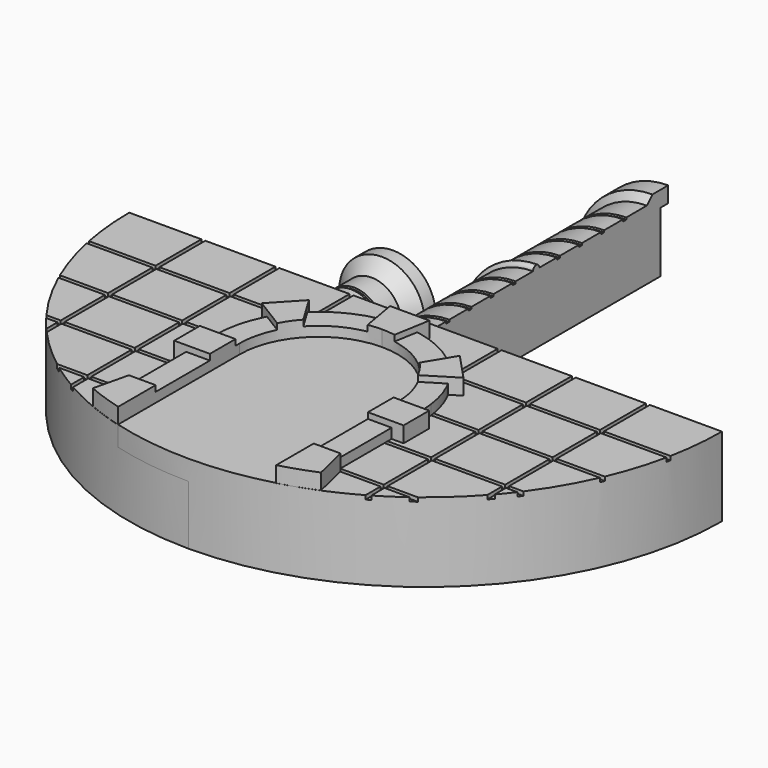
from build123d import *
from build123d import SkipClean  # not in build123d's __all__

# Parameters (mm, degrees)
F1_DEPTH  = 40
F2_W      = 36.5
F2_H      = 2
F2_W_2    = 1.9996949486
F2_W_3    = 35.5003050514
F2_W_4    = 1.9997029738
F2_W_5    = 35.5002970262
F2_W_6    = 2
F2_W_7    = 35.5
F2_H_2    = 28
F2_H_3    = 29
F2_W_8    = 1
F3_DEPTH  = 2
F5_DEPTH  = 10
F6_W      = 12
F6_H      = 12.1140629053
F6_H_2    = 4.5821502209
F7_DEPTH  = 5
F8_W      = 25.165
F8_H      = 16.205
F9_DEPTH  = 8
F10_R     = 180
F11_DEPTH = 114
F12_DEPTH = 25
F14_DEPTH = 10.1
F17_ANGLE = 90
F19_ANGLE = 180


with BuildPart() as f1:
    # F0 (on Top) → F1 (new body)
    with BuildSketch(Plane.XY):
        with BuildLine():
            Line((0, -145.5492973328), (-150, -145.5492973328))
            ThreePointArc((-150, -145.5492973328), (-106.066017178, -251.6153145107), (0, -295.5492973328))
            Line((0, -295.5492973328), (0, -145.5492973328))
        make_face()
    extrude(amount=F1_DEPTH)

    # F2 (on face) → F3 (cut)
    with BuildSketch(Plane.XY.offset(40)):
        with Locations((-131.75, -265.5492973328)):
            Rectangle(F2_W, F2_H)
        Polygon((-111.5003050514, -266.5492973328), (-113.5, -266.5492973328), (-113.5, -295.5492973328), (-111.5003050514, -295.5491274107), align=None)
        with Locations((-112.5001525257, -175.5492973328)):
            Rectangle(F2_W_2, F2_H)
        with Locations((-93.7501525257, -175.5492973328)):
            Rectangle(F2_W_3, F2_H)
        with Locations((-75.0001485131, -175.5492973328)):
            Rectangle(F2_W_4, F2_H)
        with Locations((-56.2501485131, -175.5492973328)):
            Rectangle(F2_W_5, F2_H)
        with Locations((-37.5, -175.5492973328)):
            Rectangle(F2_W_6, F2_H)
        with Locations((-18.75, -175.5492973328)):
            Rectangle(F2_W_7, F2_H)
        with Locations((-112.5001525257, -190.5492973328)):
            Rectangle(F2_W_2, F2_H_2)
        with Locations((-112.5001525257, -205.5492973328)):
            Rectangle(F2_W_2, F2_H)
        with Locations((-112.5001525257, -220.5492973328)):
            Rectangle(F2_W_2, F2_H_2)
        with Locations((-112.5001525257, -265.5492973328)):
            Rectangle(F2_W_2, F2_H)
        with Locations((-75.0001485131, -265.5492973328)):
            Rectangle(F2_W_4, F2_H)
        with Locations((-56.2501485131, -265.5492973328)):
            Rectangle(F2_W_5, F2_H)
        with Locations((-37.5, -265.5492973328)):
            Rectangle(F2_W_6, F2_H)
        with Locations((-18.75, -265.5492973328)):
            Rectangle(F2_W_7, F2_H)
        with BuildLine():
            Line((-147.1699697629, -174.5492973328), (-150, -174.5492973328))
            Line((-150, -174.5492973328), (-150, -176.5492973328))
            Line((-150, -176.5492973328), (-146.7617116281, -176.5492973328))
            ThreePointArc((-146.7617116281, -176.5492973328), (-146.9692428072, -175.5499918027), (-147.1699697629, -174.5492973328))
        make_face()
        with BuildLine():
            ThreePointArc((-137.0364914904, -206.5492973328), (-137.4765780481, -205.5508847133), (-137.9093905432, -204.5492973328))
            Line((-137.9093905432, -204.5492973328), (-150, -204.5492973328))
            Line((-150, -204.5492973328), (-150, -206.5492973328))
            Line((-150, -206.5492973328), (-137.0364914904, -206.5492973328))
        make_face()
        with BuildLine():
            ThreePointArc((-119.2434484573, -236.5492973328), (-119.9976559728, -235.5524226176), (-120.7435298474, -234.5492973328))
            Line((-120.7435298474, -234.5492973328), (-150, -234.5492973328))
            Line((-150, -234.5492973328), (-150, -236.5492973328))
            Line((-150, -236.5492973328), (-119.2434484573, -236.5492973328))
        make_face()
        Polygon((-38.5, -140.4211074114), (-38.5, -145.5492973328), (-36.5, -145.5492973328), (-36.5, -139.0285342932), align=None)
        with BuildLine():
            ThreePointArc((-36.5, -291.0407060138), (-37.5008889233, -290.7859432936), (-38.5, -290.5242951772))
            Line((-38.5, -290.5242951772), (-38.5, -295.5492973328))
            Line((-38.5, -295.5492973328), (-36.5, -295.5492973328))
            Line((-36.5, -295.5492973328), (-36.5, -291.0407060138))
        make_face()
        Polygon((-76, -139.307051897), (-76, -145.5492973328), (-74.0002970262, -145.5492973328), (-74.0002970262, -139.0285756567), align=None)
        with BuildLine():
            ThreePointArc((-74.0002970262, -276.0251803152), (-75.0023702252, -275.4517394214), (-76, -274.8706026154))
            Line((-76, -274.8706026154), (-76, -295.5492973328))
            Line((-76, -295.5492973328), (-74.0002970262, -295.5493386963))
            Line((-74.0002970262, -295.5493386963), (-74.0002970262, -276.0251803152))
        make_face()
        Polygon((-113.5, -139.307051897), (-113.5, -145.5492973328), (-111.5003050514, -145.5492973328), (-111.5003050514, -140.4209374893), align=None)
        with BuildLine():
            ThreePointArc((-111.5003050514, -245.8871365234), (-112.5058662775, -244.7583193678), (-113.5, -243.6194253025))
            Line((-113.5, -243.6194253025), (-113.5, -264.5492973328))
            Line((-113.5, -264.5492973328), (-111.5003050514, -264.5492973328))
            Line((-111.5003050514, -264.5492973328), (-111.5003050514, -245.8871365234))
        make_face()
        with BuildLine():
            Line((-91.3181252545, -264.5492973328), (-111.5003050514, -264.5492973328))
            Line((-111.5003050514, -264.5492973328), (-111.5003050514, -266.5492973328))
            Line((-111.5003050514, -266.5492973328), (-88.6510011224, -266.5492973328))
            ThreePointArc((-88.6510011224, -266.5492973328), (-89.9901195255, -265.5567070531), (-91.3181252545, -264.5492973328))
        make_face()
        with BuildLine():
            Line((-113.5, -174.5492973328), (-147.1699697629, -174.5492973328))
            ThreePointArc((-147.1699697629, -174.5492973328), (-146.9692428072, -175.5499918027), (-146.7617116281, -176.5492973328))
            Line((-146.7617116281, -176.5492973328), (-113.5, -176.5492973328))
            Line((-113.5, -176.5492973328), (-113.5, -174.5492973328))
        make_face()
        with Locations((-112.5001525257, -160.0492973328)):
            Rectangle(F2_W_2, F2_H_3)
        with Locations((-75.0001485131, -160.0492973328)):
            Rectangle(F2_W_4, F2_H_3)
        with Locations((-37.5, -160.0492973328)):
            Rectangle(F2_W_6, F2_H_3)
        with Locations((-0.5, -175.5492973328)):
            Rectangle(F2_W_8, F2_H)
        with Locations((-0.5, -190.5492973328)):
            Rectangle(F2_W_8, F2_H_2)
        with BuildLine():
            Line((-113.5, -204.5492973328), (-137.9093905432, -204.5492973328))
            ThreePointArc((-137.9093905432, -204.5492973328), (-137.4765780481, -205.5508847133), (-137.0364914904, -206.5492973328))
            Line((-137.0364914904, -206.5492973328), (-113.5, -206.5492973328))
            Line((-113.5, -206.5492973328), (-113.5, -204.5492973328))
        make_face()
        with Locations((-0.5, -205.5492973328)):
            Rectangle(F2_W_8, F2_H)
        with Locations((-0.5, -220.5492973328)):
            Rectangle(F2_W_8, F2_H_2)
        with BuildLine():
            Line((-113.5, -234.5492973328), (-120.7435298474, -234.5492973328))
            ThreePointArc((-120.7435298474, -234.5492973328), (-119.9976559728, -235.5524226176), (-119.2434484573, -236.5492973328))
            Line((-119.2434484573, -236.5492973328), (-113.5, -236.5492973328))
            Line((-113.5, -236.5492973328), (-113.5, -234.5492973328))
        make_face()
        with Locations((-0.5, -235.5492973328)):
            Rectangle(F2_W_8, F2_H)
        with BuildLine():
            Line((-111.5003050514, -236.5492973328), (-113.5, -236.5492973328))
            Line((-113.5, -236.5492973328), (-113.5, -243.6194253025))
            ThreePointArc((-113.5, -243.6194253025), (-112.5058662775, -244.7583193678), (-111.5003050514, -245.8871365234))
            Line((-111.5003050514, -245.8871365234), (-111.5003050514, -236.5492973328))
        make_face()
        with Locations((-0.5, -250.5492973328)):
            Rectangle(F2_W_8, F2_H_2)
        with BuildLine():
            Line((-76, -264.5492973328), (-91.3181252545, -264.5492973328))
            ThreePointArc((-91.3181252545, -264.5492973328), (-89.9901195255, -265.5567070531), (-88.6510011224, -266.5492973328))
            Line((-88.6510011224, -266.5492973328), (-76, -266.5492973328))
            Line((-76, -266.5492973328), (-76, -264.5492973328))
        make_face()
        with Locations((-0.5, -265.5492973328)):
            Rectangle(F2_W_8, F2_H)
        with BuildLine():
            Line((-74.0002970262, -266.5492973328), (-76, -266.5492973328))
            Line((-76, -266.5492973328), (-76, -274.8706026154))
            ThreePointArc((-76, -274.8706026154), (-75.0023702252, -275.4517394214), (-74.0002970262, -276.0251803152))
            Line((-74.0002970262, -276.0251803152), (-74.0002970262, -266.5492973328))
        make_face()
        with BuildLine():
            Line((-36.5, -266.5492973328), (-38.5, -266.5492973328))
            Line((-38.5, -266.5492973328), (-38.5, -290.5242951772))
            ThreePointArc((-38.5, -290.5242951772), (-37.5008889233, -290.7859432936), (-36.5, -291.0407060138))
            Line((-36.5, -291.0407060138), (-36.5, -266.5492973328))
        make_face()
        with Locations((-0.5, -160.0492973328)):
            Rectangle(F2_W_8, F2_H_3)
        with BuildLine():
            Line((-1, -266.5492973328), (-1, -295.5459639624))
            ThreePointArc((-1, -295.5459639624), (-0.5000027778, -295.5484639879), (0, -295.5492973328))
            Line((0, -295.5492973328), (0, -266.5492973328))
            Line((0, -266.5492973328), (-1, -266.5492973328))
        make_face()
        with BuildLine():
            Line((0, -145.5492973328), (0, -174.5492973328))
            Line((0, -174.5492973328), (0, -176.5492973328))
            Line((0, -176.5492973328), (0, -204.5492973328))
            Line((0, -204.5492973328), (0, -206.5492973328))
            Line((0, -206.5492973328), (0, -234.5492973328))
            Line((0, -234.5492973328), (0, -236.5492973328))
            Line((0, -236.5492973328), (0, -264.5492973328))
            Line((0, -264.5492973328), (0, -266.5492973328))
            Line((0, -266.5492973328), (0, -295.5492973328))
            ThreePointArc((0, -295.5492973328), (-0.5000027778, -295.5484639879), (-1, -295.5459639624))
            Line((-1, -295.5459639624), (-1, -302.514731884))
            Line((-1, -302.514731884), (2.084, -302.514731884))
            Line((2.084, -302.514731884), (2.084, -140.6996101141))
            Line((2.084, -140.6996101141), (-1, -140.6996101141))
            Line((-1, -140.6996101141), (-1, -145.5492973328))
            Line((-1, -145.5492973328), (0, -145.5492973328))
        make_face()
        with Locations((-75.0001485131, -190.5492973328)):
            Rectangle(F2_W_4, F2_H_2)
        with Locations((-93.7501525257, -205.5492973328)):
            Rectangle(F2_W_3, F2_H)
        with Locations((-56.2501485131, -205.5492973328)):
            Rectangle(F2_W_5, F2_H)
        with Locations((-37.5, -190.5492973328)):
            Rectangle(F2_W_6, F2_H_2)
        with Locations((-18.75, -205.5492973328)):
            Rectangle(F2_W_7, F2_H)
        with Locations((-18.75, -235.5492973328)):
            Rectangle(F2_W_7, F2_H)
        with Locations((-56.2501485131, -235.5492973328)):
            Rectangle(F2_W_5, F2_H)
        with Locations((-37.5, -220.5492973328)):
            Rectangle(F2_W_6, F2_H_2)
        with Locations((-37.5, -250.5492973328)):
            Rectangle(F2_W_6, F2_H_2)
        with Locations((-75.0001485131, -250.5492973328)):
            Rectangle(F2_W_4, F2_H_2)
        with Locations((-93.7501525257, -235.5492973328)):
            Rectangle(F2_W_3, F2_H)
        with Locations((-75.0001485131, -220.5492973328)):
            Rectangle(F2_W_4, F2_H_2)
        with Locations((-112.5001525257, -235.5492973328)):
            Rectangle(F2_W_2, F2_H)
        with Locations((-75.0001485131, -205.5492973328)):
            Rectangle(F2_W_4, F2_H)
        with Locations((-75.0001485131, -235.5492973328)):
            Rectangle(F2_W_4, F2_H)
        with Locations((-37.5, -205.5492973328)):
            Rectangle(F2_W_6, F2_H)
        with Locations((-37.5, -235.5492973328)):
            Rectangle(F2_W_6, F2_H)
    extrude(amount=-F3_DEPTH, mode=Mode.SUBTRACT)

    # F4 (on face) → F5 (cut)
    with BuildSketch(Plane.XY.offset(40)):
        with BuildLine():
            ThreePointArc((0, -173.1574415227), (-28.2842712475, -184.8731702752), (-40, -213.1574415227))
            Line((-40, -213.1574415227), (-40, -295.5492973328))
            Line((-40, -295.5492973328), (0, -300.0960052013))
            Line((0, -300.0960052013), (0, -173.1574415227))
        make_face()
    extrude(amount=-F5_DEPTH, mode=Mode.SUBTRACT)

    # F6 (on face) → F7 (join)
    with BuildSketch(Plane.XY.offset(40)):
        with Locations((-46, -223.9101156592)):
            Rectangle(F6_W, F6_H)
        with BuildLine():
            ThreePointArc((-46.8565880337, -190.6083803928), (-49.8587047828, -198.3889088474), (-51.5784105064, -206.5492973328))
            Line((-51.5784105064, -206.5492973328), (-39.4503793437, -206.5492973328))
            ThreePointArc((-39.4503793437, -206.5492973328), (-38.1943316303, -201.274974131), (-36.2365551908, -196.2189626092))
            Line((-36.2365551908, -196.2189626092), (-46.8565880337, -190.6083803928))
        make_face()
        with BuildLine():
            Line((-30.020735185, -186.7234584904), (-38.3793901323, -178.071512533))
            ThreePointArc((-38.3793901323, -178.071512533), (-43.0765163101, -184.0298988425), (-46.8565880337, -190.6083803928))
            Line((-46.8565880337, -190.6083803928), (-36.2365551908, -196.2189626092))
            ThreePointArc((-36.2365551908, -196.2189626092), (-33.467122398, -191.249641122), (-30.020735185, -186.7234584904))
        make_face()
        with BuildLine():
            Line((-8.9829999717, -174.1791692225), (-10.5112668126, -162.2308937309))
            ThreePointArc((-10.5112668126, -162.2308937309), (-25.6964080201, -167.9502007878), (-38.3793901323, -178.071512533))
            Line((-38.3793901323, -178.071512533), (-30.020735185, -186.7234584904))
            ThreePointArc((-30.020735185, -186.7234584904), (-20.4856690726, -178.8014032958), (-8.9829999717, -174.1791692225))
        make_face()
        with BuildLine():
            ThreePointArc((0, -173.1574415227), (3.7325532598, -173.3319717055), (7.4325343594, -173.8540392145))
            Line((7.4325343594, -173.8540392145), (7.4325343594, -161.6913611105))
            ThreePointArc((7.4325343594, -161.6913611105), (-1.5628250835, -161.1809316576), (-10.5112668126, -162.2308937309))
            Line((-10.5112668126, -162.2308937309), (-8.9829999717, -174.1791692225))
            ThreePointArc((-8.9829999717, -174.1791692225), (-4.5204594895, -173.413694266), (0, -173.1574415227))
        make_face()
        with BuildLine():
            Line((-52, -213.1574415227), (-52, -217.8530842066))
            Line((-52, -217.8530842066), (-40, -217.8530842066))
            Line((-40, -217.8530842066), (-40, -213.1574415227))
            ThreePointArc((-40, -213.1574415227), (-39.8623580195, -209.841960694), (-39.4503793437, -206.5492973328))
            Line((-39.4503793437, -206.5492973328), (-51.5784105064, -206.5492973328))
            ThreePointArc((-51.5784105064, -206.5492973328), (-51.894495596, -209.8466520649), (-52, -213.1574415227))
        make_face()
        with Locations((-46, -232.2582222223)):
            Rectangle(F6_W, F6_H_2)
        Polygon((-52, -234.5492973328), (-52, -265.6105809421), (-49.5921447873, -260.9722912312), (-40, -263.015726515), (-40, -234.5492973328), align=None)
        Polygon((-52, -265.6105809421), (-52, -296.4901937803), (-46.4878678322, -298.051148653), (-40, -284.9790668817), (-40, -263.015726515), (-49.5921447873, -260.9722912312), align=None)
        with BuildLine():
            Line((-52, -296.4901937803), (-52, -298.9768046448))
            ThreePointArc((-52, -298.9768046448), (-46.0343599341, -300.8710205574), (-40, -302.5333729583))
            Line((-40, -302.5333729583), (-40, -290.1176202808))
            Line((-40, -290.1176202808), (-40, -284.9790668817))
            Line((-40, -284.9790668817), (-46.4878678322, -298.051148653))
            Line((-46.4878678322, -298.051148653), (-52, -296.4901937803))
        make_face()
    extrude(amount=F7_DEPTH)

    # F8 (on face) → F9 (join)
    with BuildSketch(Plane.XY.offset(40)):
        Polygon((3.8162998389, -178.7047982216), (2.9556534719, -155.6107550859), (-9.9540557712, -155.6107550859), (-5.9377001598, -178.7047982216), align=None)
        Polygon((-31.0460235924, -197.7236419916), (-27.0463805646, -190.0721490383), (-38.1758213043, -171.6390103102), (-51.0442368686, -185.3769123554), align=None)
        with Locations((-45.456803869, -223.9208732462)):
            Rectangle(F8_W, F8_H)
        Polygon((-37.5396087766, -293.8241362572), (-35.3737460506, -266.3343260786), (-53.53369434, -266.3343260786), (-59.1982627344, -289.992244055), align=None)
    extrude(amount=F9_DEPTH)

    # F10 (on face) → F11 (cut)
    with BuildSketch(Plane.XY.offset(40)):
        with Locations((0, -145.5100625753)):
            Circle(F10_R)
        with BuildLine():
            Line((0, -313.7147128582), (0, -295.5100625753))
            ThreePointArc((0, -295.5100625753), (-106.066017178, -39.4440453974), (150, -145.5100625753))
            ThreePointArc((150, -145.5100625753), (112.9397266269, -244.2248950446), (20.0717580076, -294.1610784834))
            Line((20.0717580076, -294.1610784834), (19.631, -313.7147128582))
            Line((19.631, -313.7147128582), (0, -313.7147128582))
        make_face(mode=Mode.SUBTRACT)
        with BuildLine():
            Line((23.5480514792, -139.9400085211), (0, -139.9400085211))
            Line((0, -139.9400085211), (0, -295.5100625753))
            ThreePointArc((0, -295.5100625753), (10.0585191206, -295.1724365813), (20.0717580076, -294.1610784834))
            Line((20.0717580076, -294.1610784834), (23.5480514792, -139.9400085211))
        make_face()
        with BuildLine():
            ThreePointArc((20.0717580076, -294.1610784834), (10.0585191206, -295.1724365813), (0, -295.5100625753))
            Line((0, -295.5100625753), (0, -313.7147128582))
            Line((0, -313.7147128582), (19.631, -313.7147128582))
            Line((19.631, -313.7147128582), (20.0717580076, -294.1610784834))
        make_face()
    extrude(amount=F11_DEPTH, mode=Mode.SUBTRACT)

    # F12 (cut): a face of the model
    f12_faces = [f1.faces().sort_by_distance(p)[0] for p in [
        (-18.9909582241, -237.4026324516, 30),
    ]]
    extrude(f12_faces, amount=F12_DEPTH, mode=Mode.SUBTRACT)

    # F13: F1 across plane


with BuildPart() as f1_1:
    add(f1.part, clean=False)
    add(f1.part.mirror(Plane.YZ), clean=False)

    # F14 (add): a face of the model
    f14_faces = [f1_1.faces().sort_by_distance(p)[0] for p in [
        (0, -237.4026324516, 30),
    ]]
    with SkipClean():  # cleaning this boolean's faces spoils the solid; the shape is the same uncleaned
        extrude(f14_faces, amount=F14_DEPTH)

    # F16 (on Top) → F17 (revolve)
    with BuildSketch(Plane.XY):
        with BuildLine():
            Line((-35, -145.5492973328), (0, -145.5492973328))
            Line((0, -145.5492973328), (0, 2.9862365732))
            Line((0, 2.9862365732), (-30.5355339059, 2.9862365732))
            Line((-30.5355339059, 2.9862365732), (-30.5355339059, 7.9862365732))
            Line((-30.5355339059, 7.9862365732), (-38.5355339059, 7.9862365732))
            Line((-38.5355339059, 7.9862365732), (-38.5355339059, -2.0137634268))
            Line((-38.5355339059, -2.0137634268), (-35, -5.5492973328))
            Line((-35, -5.5492973328), (-35, -18.5492973328))
            Line((-35, -18.5492973328), (-34, -18.5492973328))
            Line((-34, -18.5492973328), (-34, -20.5492973328))
            Line((-34, -20.5492973328), (-35, -20.5492973328))
            Line((-35, -20.5492973328), (-35, -32.5492973328))
            Line((-35, -32.5492973328), (-34, -32.5492973328))
            Line((-34, -32.5492973328), (-34, -34.5492973328))
            Line((-34, -34.5492973328), (-35, -34.5492973328))
            Line((-35, -34.5492973328), (-35, -46.5492973328))
            Line((-35, -46.5492973328), (-34, -46.5492973328))
            Line((-34, -46.5492973328), (-34, -48.5492973328))
            Line((-34, -48.5492973328), (-35, -48.5492973328))
            Line((-35, -48.5492973328), (-35, -60.5492973328))
            Line((-35, -60.5492973328), (-34, -60.5492973328))
            Line((-34, -60.5492973328), (-34, -62.5492973328))
            Line((-34, -62.5492973328), (-35, -62.5492973328))
            Line((-35, -62.5492973328), (-35, -73.5492973328))
            ThreePointArc((-35, -73.5492973328), (-37, -75.5492973328), (-35, -77.5492973328))
            Line((-35, -77.5492973328), (-35, -88.5492973328))
            Line((-35, -88.5492973328), (-34, -88.5492973328))
            Line((-34, -88.5492973328), (-34, -90.5492973328))
            Line((-34, -90.5492973328), (-35, -90.5492973328))
            Line((-35, -90.5492973328), (-35, -102.5492973328))
            Line((-35, -102.5492973328), (-34, -102.5492973328))
            Line((-34, -102.5492973328), (-34, -104.5492973328))
            Line((-34, -104.5492973328), (-35, -104.5492973328))
            Line((-35, -104.5492973328), (-35, -116.5492973328))
            Line((-35, -116.5492973328), (-34, -116.5492973328))
            Line((-34, -116.5492973328), (-34, -118.5492973328))
            Line((-34, -118.5492973328), (-35, -118.5492973328))
            Line((-35, -118.5492973328), (-35, -130.5492973328))
            Line((-35, -130.5492973328), (-34, -130.5492973328))
            Line((-34, -130.5492973328), (-34, -132.5492973328))
            Line((-34, -132.5492973328), (-35, -132.5492973328))
            Line((-35, -132.5492973328), (-35, -145.5492973328))
        make_face()
    revolve(axis=Axis((0, -68.7815303798, 0), (0, 1, 0)), revolution_arc=F17_ANGLE)

    # F18 (on Top) → F19 (revolve)
    with BuildSketch(Plane.XY):
        Polygon((-85.5477526784, -145.5492973328), (-84.0477728305, -145.5492973328), (-70.5477526784, -145.5492973328), (-70.5477526784, -85.0154459476), (-70.5477526784, -81.5154459476), (-87.5477526784, -81.5154459476), (-87.5477526784, -78.0154459476), (-92.1167526784, -78.0154459476), (-92.1167526784, -85.0154459476), (-85.5477526784, -91.5844459476), (-85.5477526784, -102.5492973328), (-84.5477526784, -102.5492973328), (-84.5477526784, -104.5492973328), (-85.5477526784, -104.5492973328), (-85.5477526784, -116.5492973328), (-84.5477526784, -116.5492973328), (-84.5477526784, -118.5492973328), (-85.5477526784, -118.5492973328), (-85.5477526784, -130.5492973328), (-84.5477526784, -130.5492973328), (-84.5477526784, -132.5492973328), (-85.5477526784, -132.5492973328), align=None)
    revolve(axis=Axis((-70.5477526784, -115.2823716402, 0), (0, 1, 0)), revolution_arc=F19_ANGLE)


solid = f1_1.part
